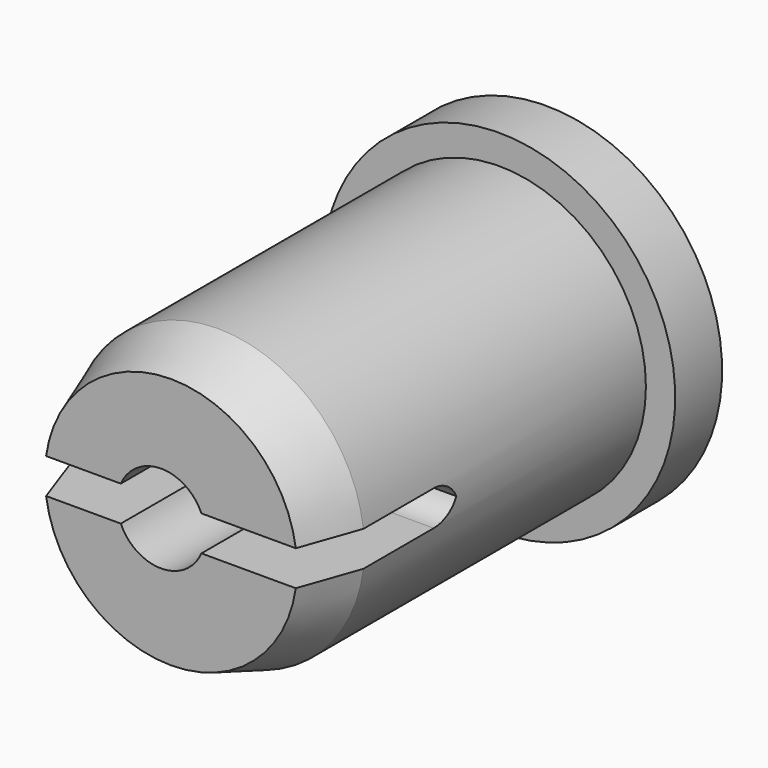
from build123d import *

# Parameters (mm, degrees)
F0_R          = 2.5
F1_DEPTH      = 6
F3_R          = 2.15
F1_FACE_R     = 2.5
F6_R          = 3
F7_DEPTH      = 1
F9_R          = 0.75
F10_DEPTH     = 8.0010001
F12_W         = 3
F12_H         = 0.3
F13_DEPTH     = 3
F14_T4_DEPTH  = 4.4618227718
F14_S5_R      = 2.5
F14_T6_DEPTH  = 4
F14_S7_R      = 0.75
F14_T8_DEPTH  = 4
F14_T12_DEPTH = 4.1272739781
F14_S13_R     = 2.5
F14_T14_DEPTH = 4
F14_S15_R     = 0.75
F14_T16_DEPTH = 4
F14_T20_DEPTH = 4.4618227718
F14_S21_R     = 2.5
F14_T22_DEPTH = 4
F14_S23_R     = 0.75
F14_T24_DEPTH = 4
F14_T28_DEPTH = 4.1272739781
F14_S29_R     = 2.5
F14_T30_DEPTH = 4
F14_S31_R     = 0.75
F14_T32_DEPTH = 4


# Not quite as in the source:
# - a fillet or chamfer that OpenCascade refuses, or shapes differently, is made with other operations: its cross-section is extruded or revolved along the edge and cut away or added


with BuildPart() as f1:
    # F0 (on Front) → F1 (new body)
    with BuildSketch(Plane.XZ):
        Circle(F0_R)
    extrude(amount=F1_DEPTH)

    # F3 (on offset) → F4 section 0
    with BuildSketch(Plane.XZ.offset(7)):
        Circle(F3_R)
    # F1_face (on face) → F4 section 1
    with BuildSketch(Plane.XZ.offset(6)):
        Circle(F1_FACE_R)
    loft()

    # F6 (on offset) → F7 (join)
    with BuildSketch(Plane(origin=(0, 0, 0), x_dir=(-1, 0, 0), z_dir=(0, 1, 0))):
        Circle(F6_R)
    extrude(amount=F7_DEPTH)

    # F9 (on offset) → F10 (cut, through all)
    with BuildSketch(Plane(origin=(0, 1, 0), x_dir=(-1, 0, 0), z_dir=(0, 1, 0))):
        with Locations((0.1672743968, 0)):
            Circle(F9_R)
    extrude(amount=-F10_DEPTH, mode=Mode.SUBTRACT)

    # F12 (on offset) → F13 (cut)
    with BuildSketch(Plane.XZ.offset(7)):
        with Locations((1.5, 0.15)):
            Rectangle(F12_W, F12_H)
        Polygon((3, 0), (0, 0), (0, 0.3), (-3, 0.3), (-3, 0), (-3, -0.3), (0, -0.3), (3, -0.3), align=None)
    extrude(amount=-F13_DEPTH, mode=Mode.SUBTRACT)

    # F14: fillet of radius 0.5 on 4 edges, made by hand


with BuildPart() as f14_tool2:
    # F14_s3 → F14_t4 (new body)
    with BuildSketch(Plane.YZ.offset(-0.7298880426)):
        with BuildLine():
            ThreePointArc((-4, 0.2), (-4.1464466094, -0.1535533906), (-4.5, -0.3))
            Line((-4.5, -0.3), (-4, -0.3))
            Line((-4, -0.3), (-4, 0.2))
        make_face()
    extrude(amount=F14_T4_DEPTH)

    # F14_s5 → F14_t6 (intersect, symmetric)
    with BuildSketch(Plane.XZ.offset(4.2)):
        Circle(F14_S5_R)
    extrude(amount=F14_T6_DEPTH, both=True, mode=Mode.INTERSECT)

    # F14_s7 → F14_t8 (cut, symmetric)
    with BuildSketch(Plane.XZ.offset(4.2)):
        with Locations((-0.1672743968, 0)):
            Circle(F14_S7_R)
    extrude(amount=F14_T8_DEPTH, both=True, mode=Mode.SUBTRACT)


with BuildPart() as f1_1:
    add(f1.part)

    # F14_t1: union F14_tool2
    add(f14_tool2.part)


with BuildPart() as f14_tool10:
    # F14_s11 → F14_t12 (new body)
    with BuildSketch(Plane.YZ.offset(-3.7319347292)):
        with BuildLine():
            ThreePointArc((-4.5, -0.3), (-4.1464466094, -0.1535533906), (-4, 0.2))
            Line((-4, 0.2), (-4, -0.3))
            Line((-4, -0.3), (-4.5, -0.3))
        make_face()
    extrude(amount=F14_T12_DEPTH)

    # F14_s13 → F14_t14 (intersect, symmetric)
    with BuildSketch(Plane.XZ.offset(4.2)):
        Circle(F14_S13_R)
    extrude(amount=F14_T14_DEPTH, both=True, mode=Mode.INTERSECT)

    # F14_s15 → F14_t16 (cut, symmetric)
    with BuildSketch(Plane.XZ.offset(4.2)):
        with Locations((-0.1672743968, 0)):
            Circle(F14_S15_R)
    extrude(amount=F14_T16_DEPTH, both=True, mode=Mode.SUBTRACT)


with BuildPart() as f1_2:
    add(f1_1.part)

    # F14_t9: union F14_tool10
    add(f14_tool10.part)


with BuildPart() as f14_tool18:
    # F14_s19 → F14_t20 (new body)
    with BuildSketch(Plane.YZ.offset(3.7319347292)):
        with BuildLine():
            ThreePointArc((-4, -0.2), (-4.1464466094, 0.1535533906), (-4.5, 0.3))
            Line((-4.5, 0.3), (-4, 0.3))
            Line((-4, 0.3), (-4, -0.2))
        make_face()
    extrude(amount=-F14_T20_DEPTH)

    # F14_s21 → F14_t22 (intersect, symmetric)
    with BuildSketch(Plane.XZ.offset(4.2)):
        Circle(F14_S21_R)
    extrude(amount=F14_T22_DEPTH, both=True, mode=Mode.INTERSECT)

    # F14_s23 → F14_t24 (cut, symmetric)
    with BuildSketch(Plane.XZ.offset(4.2)):
        with Locations((-0.1672743968, 0)):
            Circle(F14_S23_R)
    extrude(amount=F14_T24_DEPTH, both=True, mode=Mode.SUBTRACT)


with BuildPart() as f1_3:
    add(f1_2.part)

    # F14_t17: union F14_tool18
    add(f14_tool18.part)


with BuildPart() as f14_tool26:
    # F14_s27 → F14_t28 (new body)
    with BuildSketch(Plane.YZ.offset(0.3953392489)):
        with BuildLine():
            ThreePointArc((-4, -0.2), (-4.1464466094, 0.1535533906), (-4.5, 0.3))
            Line((-4.5, 0.3), (-4, 0.3))
            Line((-4, 0.3), (-4, -0.2))
        make_face()
    extrude(amount=-F14_T28_DEPTH)

    # F14_s29 → F14_t30 (intersect, symmetric)
    with BuildSketch(Plane.XZ.offset(4.2)):
        Circle(F14_S29_R)
    extrude(amount=F14_T30_DEPTH, both=True, mode=Mode.INTERSECT)

    # F14_s31 → F14_t32 (cut, symmetric)
    with BuildSketch(Plane.XZ.offset(4.2)):
        with Locations((-0.1672743968, 0)):
            Circle(F14_S31_R)
    extrude(amount=F14_T32_DEPTH, both=True, mode=Mode.SUBTRACT)


with BuildPart() as f1_4:
    add(f1_3.part)

    # F14_t25: union F14_tool26
    add(f14_tool26.part)


solid = f1_4.part
